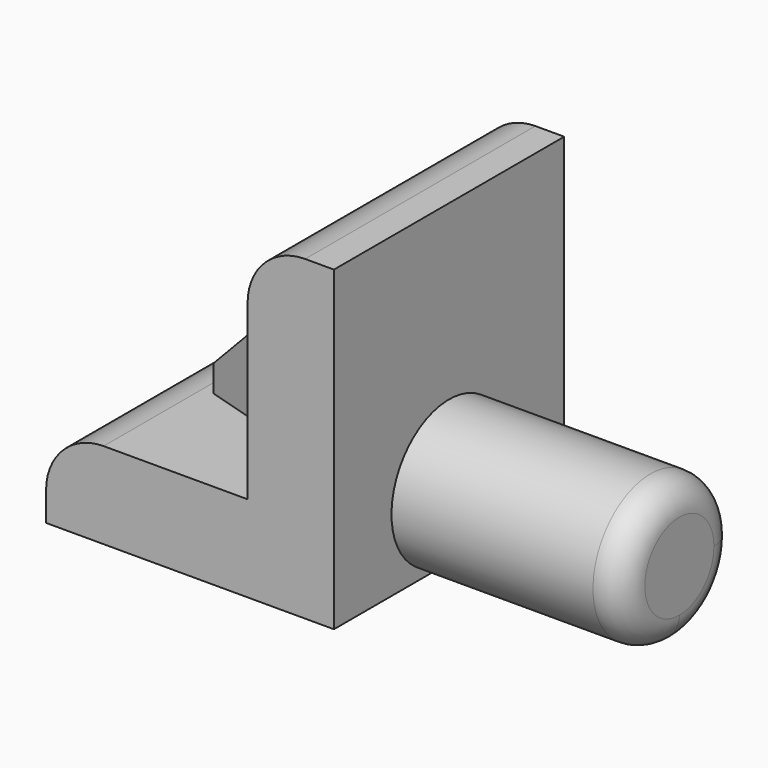
from build123d import *

# Parameters (mm, degrees)
F0_W        = 10
F0_H        = 10
F1_DEPTH    = 3
F3_DEPTH    = 8
F4_DEPTH    = 6
F5_T4_DEPTH = 27.5665061863
F6_R        = 2
F8_DEPTH    = 8
F9_R        = 1


# Not quite as in the source:
# - a fillet or chamfer that OpenCascade refuses, or shapes differently, is made with other operations: its cross-section is extruded or revolved along the edge and cut away or added


with BuildPart() as f1:
    # F0 (on Top) → F1 (new body)
    with BuildSketch(Plane.XY):
        with Locations((-5, -7.9495952278)):
            Rectangle(F0_W, F0_H)
    extrude(amount=F1_DEPTH)

    # F2 (on face) → F3 (join)
    with BuildSketch(Plane.XY.offset(3)):
        Polygon((0, -12.9495952278), (0, -2.9495952278), (-3, -2.9495952278), (-3, -5.8524622582), (-3, -7.9495952278), (-3, -10.0610805675), (-3, -12.9495952278), align=None)
    extrude(amount=F3_DEPTH)

    # F2 (on face) → F4 (join)
    with BuildSketch(Plane.XY.offset(3)):
        Polygon((-3, -7.9495952278), (-3, -5.8524622582), (-7.6078968298, -7.2329440242), (-7.6078968298, -8.6711510528), (-3, -10.0610805675), align=None)
    extrude(amount=F4_DEPTH)

    # F5: chamfer of 5.08 on 1 edges, made by hand


with BuildPart() as f5_tool2:
    # F5_s3 → F5_t4 (new body)
    with BuildSketch(Plane.XZ.offset(-5.8312055546)):
        Polygon((-7.6078968298, 3.92), (-2.5278968298, 9), (-7.6078968298, 9), align=None)
    extrude(amount=F5_T4_DEPTH)

    split(bisect_by=Plane.YZ.offset(-3), keep=Keep.BOTTOM)


with BuildPart() as f1_1:
    add(f1.part)

    # F5_t1: cut F5_tool2
    add(f5_tool2.part, mode=Mode.SUBTRACT)

    # F6
    f6_edges = [f1_1.edges().sort_by_distance(p)[0] for p in [
        (-10, -7.949595, 3),
        (-3, -7.949595, 11),
    ]]
    fillet(f6_edges, radius=F6_R)

    # F7 (on face) → F8 (join)
    with BuildSketch(Plane.YZ):
        with BuildLine():
            ThreePointArc((-7.9495952278, 0), (-6.1818282749, 0.732233047), (-5.4495952278, 2.5))
            ThreePointArc((-5.4495952278, 2.5), (-9.7173621808, 4.267766953), (-7.9495952278, 0))
        make_face()
    extrude(amount=F8_DEPTH)

    # F9
    f9_edges = [f1_1.edges().sort_by_distance(p)[0] for p in [
        (8, -7.949595, 5),
    ]]
    fillet(f9_edges, radius=F9_R)


solid = f1_1.part
